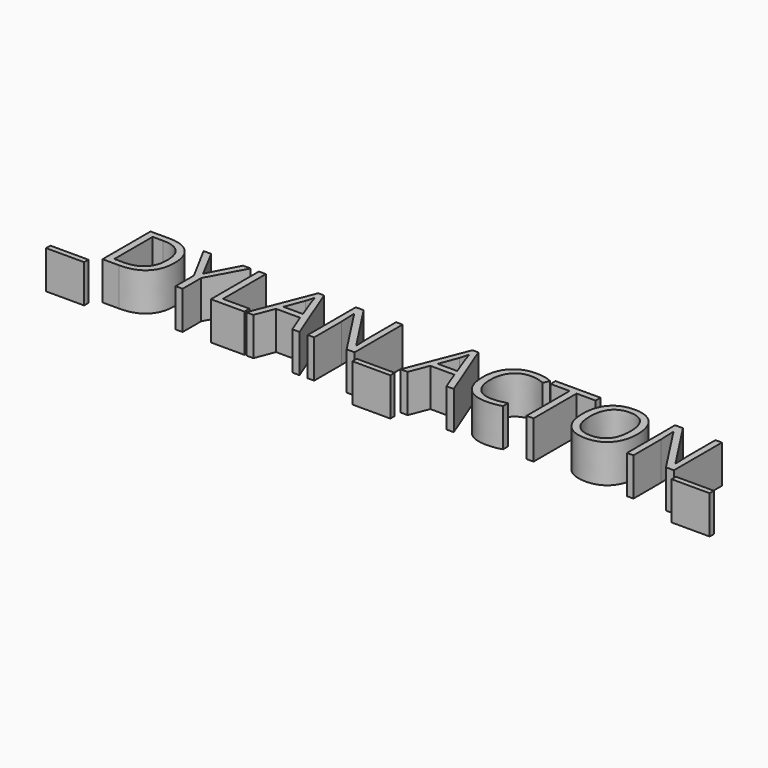
from build123d import *

# Parameters (mm, degrees)
F0_TEXT_SIZE = 55.1437292921
F1_DEPTH     = 25


# Not quite as in the source:
# - Text() gives the source's letters only with a copy of the font that has no kerning and outlines rounded to 1/6400 em; it was checked with that copy


with BuildPart() as f1:
    # F0 (on Top) → F1 (new body)
    with BuildSketch(Plane.XY):
        with Locations((-181.8185038865, 3.2411958091)):
            Text('_DYLAN_ACTON_', F0_TEXT_SIZE, font='Open Sans', text_align=(TextAlign.LEFT, TextAlign.BOTTOM))
    extrude(amount=F1_DEPTH)


solid = f1.part
